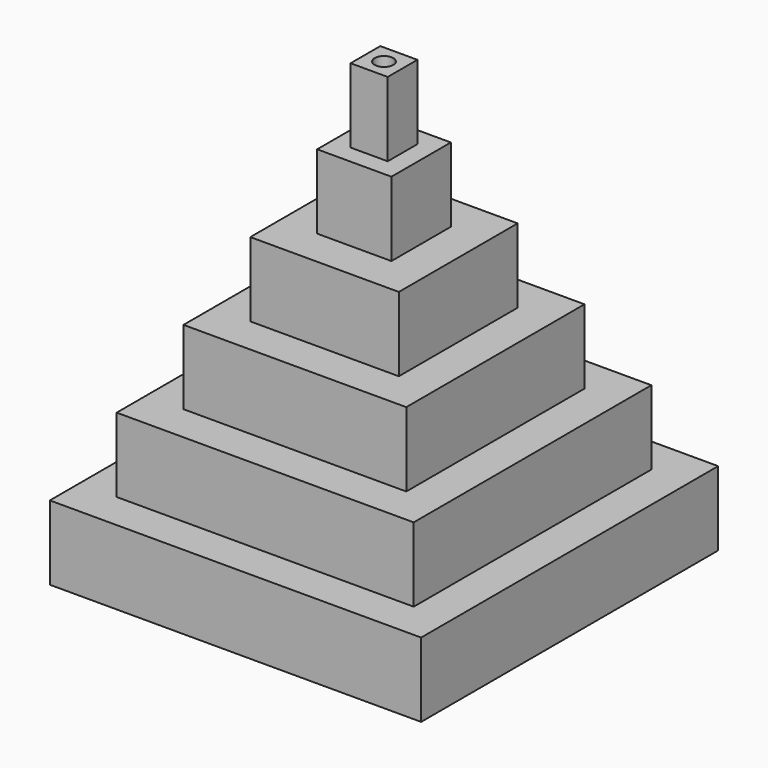
from build123d import *

# Parameters (mm, degrees)
F0_W     = 127
F0_H     = 127
F0_W_2   = 101.6
F0_H_2   = 101.6
F1_DEPTH = 25.4
F0_W_3   = 76.2
F0_H_3   = 76.2
F2_DEPTH = 50.8
F0_W_4   = 50.8
F0_H_4   = 50.8
F3_DEPTH = 76.2
F0_W_5   = 25.4
F0_H_5   = 25.4
F4_DEPTH = 101.6
F0_W_6   = 12.7
F0_H_6   = 12.7
F5_DEPTH = 127
F0_R     = 3.175
F6_DEPTH = 152.4


# Not quite as in the source:
# - the program builds the solid bodies; features that only make, move or delete a surface that nothing else refers to are left out


with BuildPart() as f1:
    # F0 (on Top) → F1 (new body)
    with BuildSketch(Plane.XY):
        Rectangle(F0_W, F0_H)
        Rectangle(F0_W_2, F0_H_2, mode=Mode.SUBTRACT)
    extrude(amount=F1_DEPTH)


with BuildPart() as f2:
    # F0 (on Top) → F2 (new body)
    with BuildSketch(Plane.XY):
        Rectangle(F0_W_2, F0_H_2)
        Rectangle(F0_W_3, F0_H_3, mode=Mode.SUBTRACT)
    extrude(amount=F2_DEPTH)


with BuildPart() as f3:
    # F0 (on Top) → F3 (new body)
    with BuildSketch(Plane.XY):
        Rectangle(F0_W_3, F0_H_3)
        Rectangle(F0_W_4, F0_H_4, mode=Mode.SUBTRACT)
    extrude(amount=F3_DEPTH)


with BuildPart() as f4:
    # F0 (on Top) → F4 (new body)
    with BuildSketch(Plane.XY):
        Rectangle(F0_W_4, F0_H_4)
        Rectangle(F0_W_5, F0_H_5, mode=Mode.SUBTRACT)
    extrude(amount=F4_DEPTH)


with BuildPart() as f5:
    # F0 (on Top) → F5 (new body)
    with BuildSketch(Plane.XY):
        Rectangle(F0_W_5, F0_H_5)
        Rectangle(F0_W_6, F0_H_6, mode=Mode.SUBTRACT)
    extrude(amount=F5_DEPTH)


with BuildPart() as f6:
    # F0 (on Top) → F6 (new body)
    with BuildSketch(Plane.XY):
        Rectangle(F0_W_6, F0_H_6)
        Circle(F0_R, mode=Mode.SUBTRACT)
    extrude(amount=F6_DEPTH)


solid = Compound([f1.part, f2.part, f3.part, f4.part, f5.part, f6.part])
